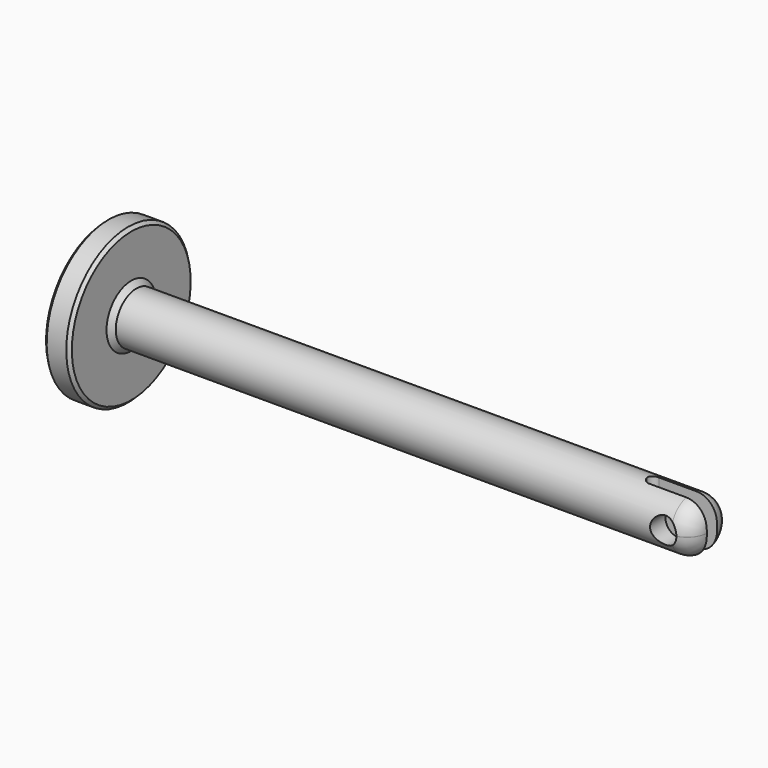
from build123d import *

# Parameters (mm, degrees)
F0_W        = 143
F0_H        = 6.35
F2_SIZE     = 0.762
F3_SIZE     = 1.27
F4_R        = 3.175
F5_DEPTH    = 12.7
F6_W        = 15.875
F6_H        = 3.175
F7_DEPTH    = 12.7
F8_R        = 1.5874
F9_T2_ANGLE = 359.64
F9_T4_ANGLE = 359.64


# Not quite as in the source:
# - a fillet or chamfer that OpenCascade refuses, or shapes differently, is made with other operations: its cross-section is extruded or revolved along the edge and cut away or added
# - a fillet or chamfer is up to 0.001 mm smaller than in the source, because OpenCascade refuses the exact size


with BuildPart() as f1:
    # F0 (on Front) → F1 (revolve)
    with BuildSketch(Plane.XZ):
        Polygon((0, 19.05), (-6.35, 19.05), (-6.35, 0), (0, 0), (0, 6.35), align=None)
        with Locations((71.5, 3.175)):
            Rectangle(F0_W, F0_H)
    revolve(axis=Axis((71.5, 0, 0), (1, 0, 0)))

    # F2
    f2_edges = [f1.edges().sort_by_distance(p)[0] for p in [
        (0, 0, -19.05),
        (-6.35, 0, -19.05),
    ]]
    chamfer(f2_edges, length=F2_SIZE)

    # F3
    f3_edges = [f1.edges().sort_by_distance(p)[0] for p in [
        (0, 0, -6.35),
    ]]
    chamfer(f3_edges, length=F3_SIZE)

    # F4 (on Front) → F5 (cut, symmetric)
    with BuildSketch(Plane.XZ):
        with Locations((136, 0)):
            Circle(F4_R)
    extrude(amount=F5_DEPTH, both=True, mode=Mode.SUBTRACT)

    # F6 (on Top) → F7 (cut, symmetric)
    with BuildSketch(Plane.XY):
        with Locations((135.0625, 0)):
            Rectangle(F6_W, F6_H)
    extrude(amount=F7_DEPTH, both=True, mode=Mode.SUBTRACT)

    # F8 (radius 1.5875 in the source; OpenCascade refuses exactly that, so slightly less here)
    f8_edges = [f1.edges().sort_by_distance(p)[0] for p in [
        (127.125, 1.5875, 0),
        (127.125, -1.5875, 0),
    ]]
    fillet(f8_edges, radius=F8_R)

    # F9: fillet of radius 5.08 on 2 edges, made by hand

    # F9_s1 → F9_t2 (revolve, cut)
    with BuildSketch(Plane(origin=(0, 0, 0), x_dir=(1, 0, 0), z_dir=(0, -0.0031415875, 0.9999950652))):
        with BuildLine():
            ThreePointArc((137.92, -6.35), (141.5121024484, -4.8621024484), (143, -1.27))
            Line((143, -1.27), (143, -6.35))
            Line((143, -6.35), (137.92, -6.35))
        make_face()
    revolve(axis=Axis((143, 0, 0), (1, 0, 0)), revolution_arc=F9_T2_ANGLE, mode=Mode.SUBTRACT)

    # F9_s3 → F9_t4 (revolve, cut)
    with BuildSketch(Plane(origin=(0, 0, 0), x_dir=(1, 0, 0), z_dir=(0, 0.0031415875, -0.9999950652))):
        with BuildLine():
            ThreePointArc((137.92, -6.35), (141.5121024484, -4.8621024484), (143, -1.27))
            Line((143, -1.27), (143, -6.35))
            Line((143, -6.35), (137.92, -6.35))
        make_face()
    revolve(axis=Axis((143, 0, 0), (1, 0, 0)), revolution_arc=F9_T4_ANGLE, mode=Mode.SUBTRACT)


solid = f1.part
